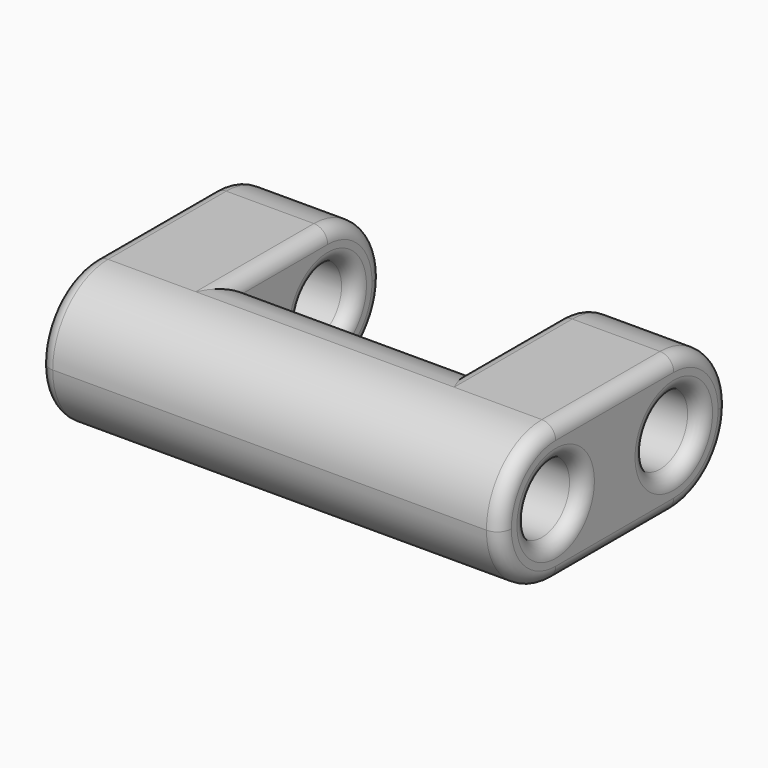
from build123d import *

# Parameters (mm, degrees)
F1_DEPTH = 7.62
F2_R     = 3.80999
F3_R     = 1.905
F4_DEPTH = 25.4
F5_R     = 0.762


# Not quite as in the source:
# - a fillet or chamfer is up to 0.001 mm smaller than in the source, because OpenCascade refuses the exact size


with BuildPart() as f1:
    # F0 (on Top) → F1 (new body)
    with BuildSketch(Plane.XY):
        Polygon((0, 15.748), (0, 0), (25.4, 0), (25.4, 15.748), (19.05, 15.748), (19.05, 7.62), (6.35, 7.62), (6.35, 15.748), align=None)
    extrude(amount=F1_DEPTH)

    # F2 (radius 3.81 in the source; OpenCascade refuses exactly that, so slightly less here)
    f2_edges = [f1.edges().sort_by_distance(p)[0] for p in [
        (12.7, 0, 7.62),
        (12.7, 0, 0),
        (22.225, 15.748, 7.62),
        (22.225, 15.748, 0),
        (12.7, 7.62, 7.62),
        (12.7, 7.62, 0),
        (3.175, 15.748, 7.62),
        (3.175, 15.748, 0),
    ]]
    fillet(f2_edges, radius=F2_R)

    # F3 (on face) → F4 (cut)
    with BuildSketch(Plane.YZ.offset(25.4)):
        with Locations((3.81, 3.81)):
            Circle(F3_R)
        with Locations((11.938, 3.81)):
            Circle(F3_R)
    extrude(amount=-F4_DEPTH, mode=Mode.SUBTRACT)

    # F5
    f5_edges = [f1.edges().sort_by_distance(p)[0] for p in [
        (25.4, 0, 3.81),
        (25.4, 1.11592, 1.11592),
        (25.4, 1.11592, 6.50408),
        (25.4, 7.874, 0),
        (25.4, 7.874, 7.62),
        (25.4, 14.63208, 1.11592),
        (25.4, 14.63208, 6.50408),
        (25.4, 15.748, 3.81),
        (25.4, 10.033, 3.81),
        (25.4, 1.905, 3.81),
        (0, 15.748, 3.81),
        (0, 14.63208, 1.11592),
        (0, 14.63208, 6.50408),
        (0, 7.874, 0),
        (0, 7.874, 7.62),
        (0, 1.11592, 1.11592),
        (0, 1.11592, 6.50408),
        (0, 0, 3.81),
        (0, 10.033, 3.81),
        (0, 1.905, 3.81),
        (6.35, 14.63208, 1.11592),
        (6.35, 10.033, 3.81),
        (19.05, 10.033, 3.81),
        (19.05, 14.63208, 1.11592),
    ]]
    fillet(f5_edges, radius=F5_R)


solid = f1.part
